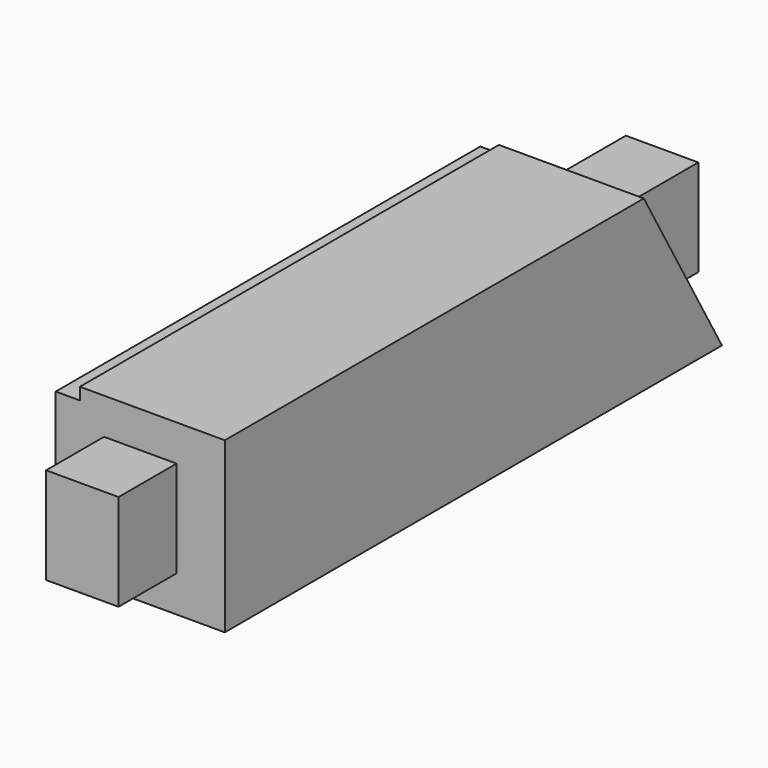
from build123d import *

# Parameters (mm, degrees)
F0_W     = 381
F0_H     = 88.9
F1_DEPTH = 44.45
F5_W     = 12.7
F5_H     = 6.35
F6_DEPTH = 381.001
F4_W     = 88.9
F4_H     = 88.9
F4_W_2   = 38.1
F4_H_2   = 50.8
F7_REACH = 193.287585695
F8_W     = 88.9
F8_H     = 88.9
F8_W_2   = 38.1
F8_H_2   = 50.8
F9_DEPTH = 38.1


with BuildPart() as f1:
    # F0 (on Right) → F1 (new body, symmetric)
    with BuildSketch(Plane.YZ):
        Rectangle(F0_W, F0_H)
    extrude(amount=F1_DEPTH, both=True)

    # F5 (on face) → F6 (cut, through all)
    with BuildSketch(Plane(origin=(0, 190.5, 0), x_dir=(-1, 0, 0), z_dir=(0, 1, 0))):
        with Locations((38.1, 41.275)):
            Rectangle(F5_W, F5_H)
    extrude(amount=-F6_DEPTH, mode=Mode.SUBTRACT)

    f7_end = Plane(origin=(0, 111.4494145991, 64.3453495198), x_dir=(0, 0.5, -0.8660254038), z_dir=(0, -0.8660254038, -0.5))
    # F4 (on face) → F7 (cut, up to a plane its end follows)
    with BuildSketch(Plane(origin=(0, 190.5, 0), x_dir=(-1, 0, 0), z_dir=(0, 1, 0))):
        Rectangle(F4_W, F4_H)
        Rectangle(F4_W_2, F4_H_2, mode=Mode.SUBTRACT)
    f7_long = extrude(amount=-F7_REACH, mode=Mode.PRIVATE)
    add(split(f7_long, bisect_by=f7_end, keep=Keep.BOTTOM, mode=Mode.PRIVATE), mode=Mode.SUBTRACT)

    # F8 (on face) → F9 (cut)
    with BuildSketch(Plane.XZ.offset(190.5)):
        Rectangle(F8_W, F8_H)
        Rectangle(F8_W_2, F8_H_2, mode=Mode.SUBTRACT)
    extrude(amount=-F9_DEPTH, mode=Mode.SUBTRACT)


solid = f1.part
